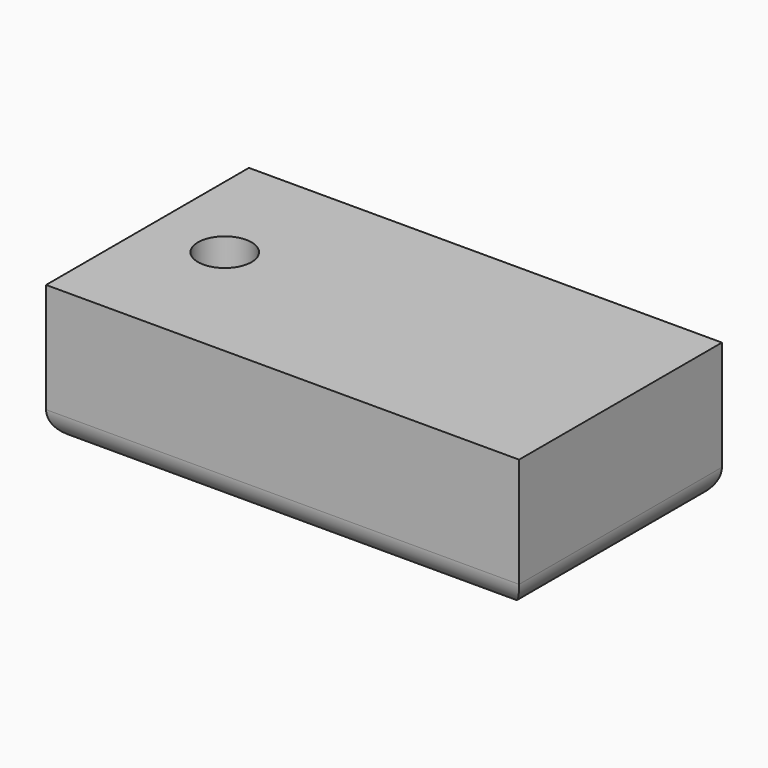
from build123d import *

# Parameters (mm, degrees)
F0_W        = 87.5617265701
F0_H        = 46.9353795052
F1_DEPTH    = 25.4
F2_R        = 4.9619580549
F3_DEPTH    = 25.4
F4_T1_DEPTH = 72.3353795052
F4_T3_DEPTH = 112.9617265701


# Not quite as in the source:
# - a fillet or chamfer that OpenCascade refuses, or shapes differently, is made with other operations: its cross-section is extruded or revolved along the edge and cut away or added


with BuildPart() as f1:
    # F0 (on Top) → F1 (new body)
    with BuildSketch(Plane.XY):
        with Locations((43.7808632851, 23.4676897526)):
            Rectangle(F0_W, F0_H)
    extrude(amount=F1_DEPTH)

    # F2 (on face) → F3 (cut)
    with BuildSketch(Plane.XY.offset(25.4)):
        with Locations((13.7676307932, 24.1377800703)):
            Circle(F2_R)
    extrude(amount=-F3_DEPTH, mode=Mode.SUBTRACT)

    # F4: fillet of radius 5.08 on 5 edges, made by hand

    # F4_s2 → F4_t1 (cut)
    with BuildSketch(Plane.XZ.offset(-59.6353795052)):
        with BuildLine():
            ThreePointArc((0, 5.08), (1.4878975516, 1.4878975516), (5.08, 0))
            Line((5.08, 0), (0, 0))
            Line((0, 0), (0, 5.08))
        make_face()
        with BuildLine():
            ThreePointArc((82.4817265701, 0), (86.0738290186, 1.4878975516), (87.5617265701, 5.08))
            Line((87.5617265701, 5.08), (87.5617265701, 0))
            Line((87.5617265701, 0), (82.4817265701, 0))
        make_face()
    extrude(amount=F4_T1_DEPTH, mode=Mode.SUBTRACT)

    # F4_s4 → F4_t3 (cut)
    with BuildSketch(Plane.YZ.offset(-12.7)):
        with BuildLine():
            ThreePointArc((46.9353795052, 5.08), (45.4474819536, 1.4878975516), (41.8553795052, 0))
            Line((41.8553795052, 0), (46.9353795052, 0))
            Line((46.9353795052, 0), (46.9353795052, 5.08))
        make_face()
        with BuildLine():
            ThreePointArc((0, 5.08), (1.4878975516, 1.4878975516), (5.08, 0))
            Line((5.08, 0), (0, 0))
            Line((0, 0), (0, 5.08))
        make_face()
    extrude(amount=F4_T3_DEPTH, mode=Mode.SUBTRACT)

    # F4_s5 → F4_t6 (revolve, cut)
    with BuildSketch(Plane.XZ.offset(-24.1377800703)):
        with BuildLine():
            ThreePointArc((23.809588848, 0), (20.2174863996, 1.4878975516), (18.729588848, 5.08))
            Line((18.729588848, 5.08), (18.729588848, 0))
            Line((18.729588848, 0), (23.809588848, 0))
        make_face()
    revolve(axis=Axis((13.7676307932, 24.1377800703, 0), (0, 0, 1)), mode=Mode.SUBTRACT)


solid = f1.part
